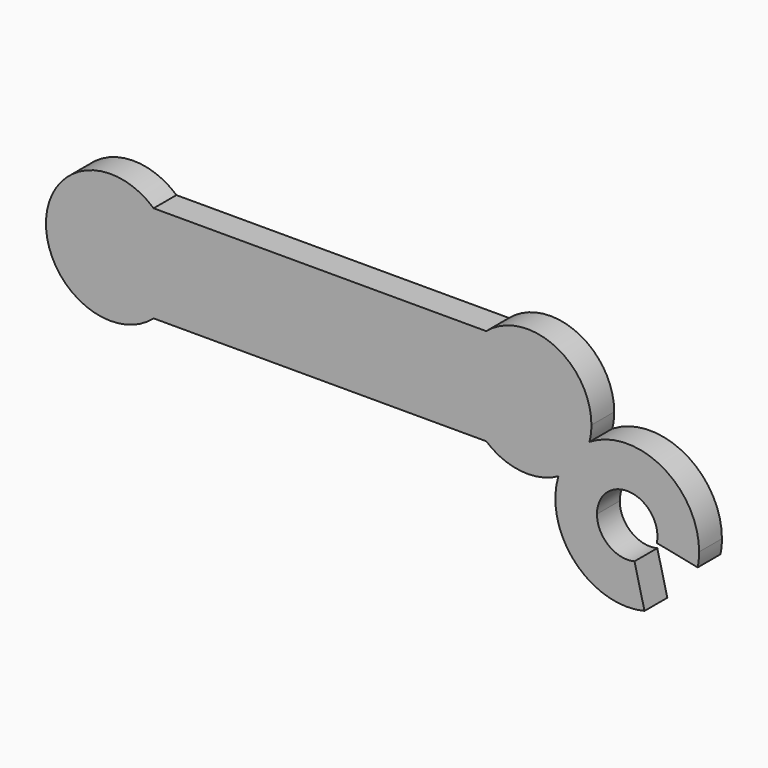
from build123d import *

# Parameters (mm, degrees)
F1_DEPTH = 3
F3_DEPTH = 25


# Not quite as in the source:
# - a feature names something its author has since deleted; it is built from what else it names


with BuildPart() as f1:
    # F0 (on Front) → F1 (new body)
    with BuildSketch(Plane.XZ):
        with BuildLine():
            Line((-24.6447846293, -46.4568324387), (-24.6447846293, -56.6546805203))
            Line((-24.6447846293, -56.6546805203), (-23.8253123528, -56.6546805203))
            ThreePointArc((-23.8253123528, -56.6546805203), (-22.130084006, -54.3516793641), (-21.5297268649, -51.5557564795))
            ThreePointArc((-21.5297268649, -51.5557564795), (-22.130084006, -48.7598335949), (-23.8253123528, -46.4568324387))
            Line((-23.8253123528, -46.4568324387), (-24.6447846293, -46.4568324387))
        make_face()
        with BuildLine():
            Line((-23.8253123528, -56.6546805203), (-24.6447846293, -56.6546805203))
            Line((-24.6447846293, -56.6546805203), (-24.6447846293, -46.4568324387))
            Line((-24.6447846293, -46.4568324387), (-23.8253123528, -46.4568324387))
            ThreePointArc((-23.8253123528, -46.4568324387), (-35.1509748081, -51.5557564795), (-23.8253123528, -56.6546805203))
        make_face()
        with BuildLine():
            ThreePointArc((-21.5297268649, -51.5557564795), (-22.130084006, -54.3516793641), (-23.8253123528, -56.6546805203))
            Line((-23.8253123528, -56.6546805203), (11.1679025889, -56.6546805203))
            ThreePointArc((11.1679025889, -56.6546805203), (8.8185102803, -51.5557564795), (11.1679025889, -46.4568324387))
            Line((11.1679025889, -46.4568324387), (-23.8253123528, -46.4568324387))
            ThreePointArc((-23.8253123528, -46.4568324387), (-22.130084006, -48.7598335949), (-21.5297268649, -51.5557564795))
        make_face()
        with BuildLine():
            ThreePointArc((11.1679025889, -46.4568324387), (8.8185102803, -51.5557564795), (11.1679025889, -56.6546805203))
            Line((11.1679025889, -56.6546805203), (11.8974819779, -56.6546805203))
            Line((11.8974819779, -56.6546805203), (11.8974819779, -46.4568324387))
            Line((11.8974819779, -46.4568324387), (11.1679025889, -46.4568324387))
        make_face()
        with BuildLine():
            Line((11.8974819779, -56.6546805203), (11.1679025889, -56.6546805203))
            ThreePointArc((11.1679025889, -56.6546805203), (14.8431416467, -58.2287078356), (18.7610955863, -57.4321018799))
            ThreePointArc((18.7610955863, -57.4321018799), (20.0078661899, -55.0037023767), (22.0355331957, -53.1761007794))
            ThreePointArc((22.0355331957, -53.1761007794), (22.1843328788, -52.371994204), (22.234179719, -51.5557564795))
            ThreePointArc((22.234179719, -51.5557564795), (18.3334195709, -45.4635172382), (11.1679025889, -46.4568324387))
            Line((11.1679025889, -46.4568324387), (11.8974819779, -46.4568324387))
            Line((11.8974819779, -46.4568324387), (11.8974819779, -56.6546805203))
        make_face()
        with BuildLine():
            ThreePointArc((22.0355331957, -53.1761007794), (20.0078661899, -55.0037023767), (18.7610955863, -57.4321018799))
            ThreePointArc((18.7610955863, -57.4321018799), (20.8427791516, -55.6460589781), (22.0355331957, -53.1761007794))
        make_face()
        with BuildLine():
            ThreePointArc((22.0355331957, -53.1761007794), (20.8427791516, -55.6460589781), (18.7610955863, -57.4321018799))
            ThreePointArc((18.7610955863, -57.4321018799), (24.8985692809, -67.0974714468), (33.5650116518, -59.615444392))
            ThreePointArc((33.5650116518, -59.615444392), (29.6898526428, -53.0125279979), (22.0355331957, -53.1761007794))
        make_face()
    extrude(amount=F1_DEPTH)

    # F2 (on face) → F3 (cut)
    with BuildSketch(Plane(origin=(0, 0, 0), x_dir=(-1, 0, 0), z_dir=(0, 1, 0))):
        with BuildLine():
            ThreePointArc((-26.7674391798, -62.7047392847), (-28.3016132323, -61.8158013566), (-29.1220744495, -60.2439412946))
            Line((-29.1220744495, -60.2439412946), (-33.4160842435, -61.108925342))
            ThreePointArc((-33.4160842435, -61.108925342), (-31.4664434529, -64.8440957921), (-27.8208252933, -66.9564560213))
            Line((-27.8208252933, -66.9564560213), (-26.7674391798, -62.7047392847))
        make_face()
        with BuildLine():
            ThreePointArc((-27.8208252933, -66.9564560213), (-31.4664434529, -64.8440957921), (-33.4160842435, -61.108925342))
            Line((-33.4160842435, -61.108925342), (-39.6901629865, -62.3727738857))
            Line((-39.6901629865, -62.3727738857), (-29.0901046246, -72.0795691013))
            Line((-29.0901046246, -72.0795691013), (-27.8208252933, -66.9564560213))
        make_face()
        with BuildLine():
            Line((-26.0020494461, -59.615444392), (-29.1220744495, -60.2439412946))
            ThreePointArc((-29.1220744495, -60.2439412946), (-28.3016132323, -61.8158013566), (-26.7674391798, -62.7047392847))
            Line((-26.7674391798, -62.7047392847), (-26.0020494461, -59.615444392))
        make_face()
        with BuildLine():
            ThreePointArc((-26.7674391798, -62.7047392847), (-24.0407284287, -62.1219926651), (-22.8193517887, -59.615444392))
            ThreePointArc((-22.8193517887, -59.615444392), (-26.3178564355, -56.4484536556), (-29.1220744495, -60.2439412946))
            Line((-29.1220744495, -60.2439412946), (-26.0020494461, -59.615444392))
            Line((-26.0020494461, -59.615444392), (-26.7674391798, -62.7047392847))
        make_face()
    extrude(amount=-F3_DEPTH, mode=Mode.SUBTRACT)


solid = f1.part
